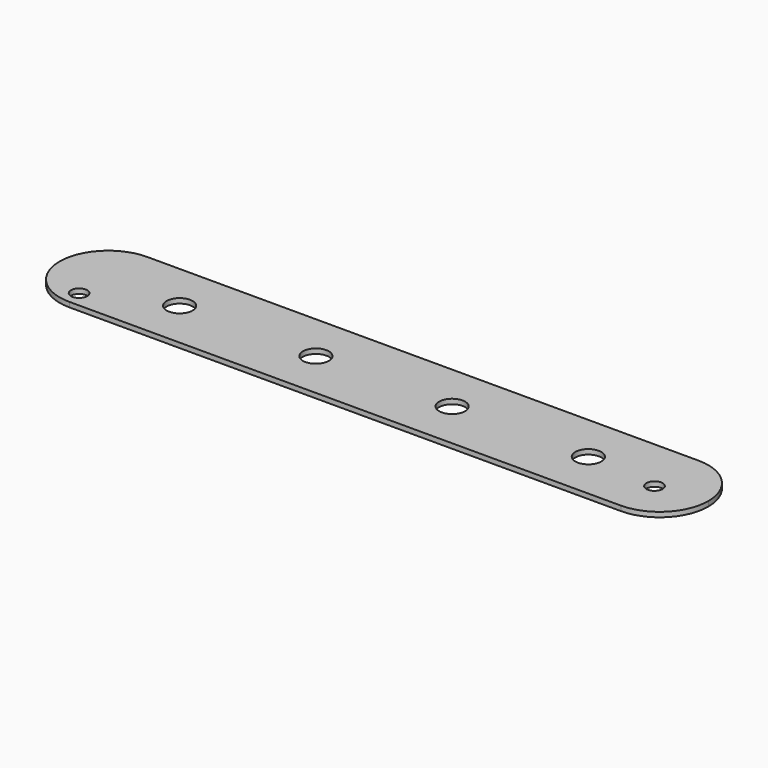
from build123d import *

# Parameters (mm, degrees)
F0_W     = 200
F0_H     = 30
F0_R     = 2.5
F0_R_2   = 4
F1_DEPTH = 1.5
F2_R     = 14.99999


# Not quite as in the source:
# - a fillet or chamfer is up to 0.001 mm smaller than in the source, because OpenCascade refuses the exact size


with BuildPart() as f1:
    # F0 (on Top) → F1 (new body)
    with BuildSketch(Plane.XY):
        Rectangle(F0_W, F0_H)
        with Locations((-86, -10)):
            Circle(F0_R, mode=Mode.SUBTRACT)
        with Locations((85, -2)):
            Circle(F0_R, mode=Mode.SUBTRACT)
        with Locations((-63, 0)):
            Circle(F0_R_2, mode=Mode.SUBTRACT)
        with Locations((-21, 0)):
            Circle(F0_R_2, mode=Mode.SUBTRACT)
        with Locations((21, 0)):
            Circle(F0_R_2, mode=Mode.SUBTRACT)
        with Locations((63, 0)):
            Circle(F0_R_2, mode=Mode.SUBTRACT)
    extrude(amount=F1_DEPTH)

    # F2 (radius 15 in the source; OpenCascade refuses exactly that, so slightly less here)
    f2_edges = [f1.edges().sort_by_distance(p)[0] for p in [
        (-100, -15, 0.75),
        (-100, 15, 0.75),
        (100, -15, 0.75),
        (100, 15, 0.75),
    ]]
    fillet(f2_edges, radius=F2_R)


solid = f1.part
